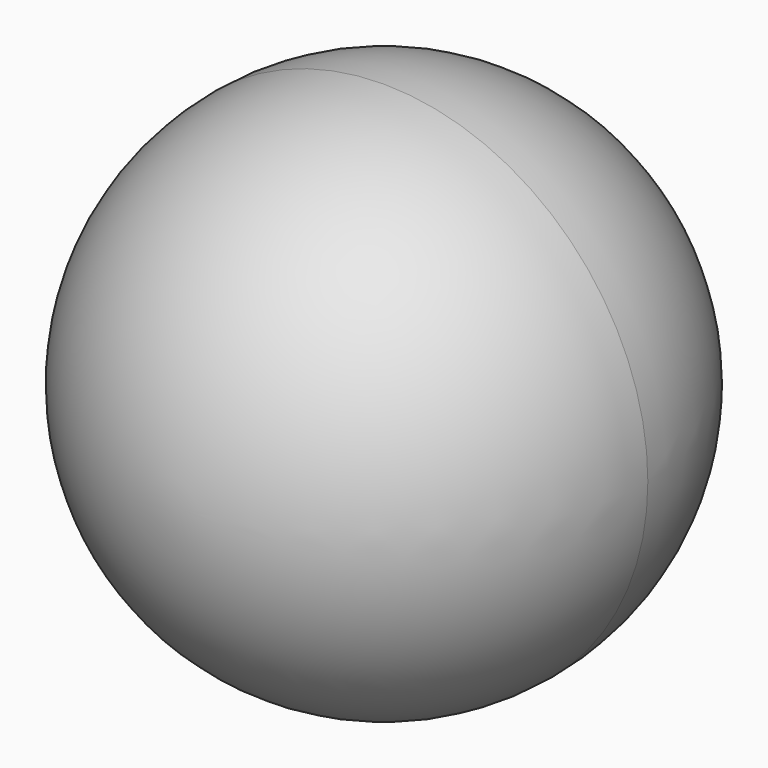
from build123d import *


with BuildPart() as f1:
    # F0 (on Top) → F1 (revolve)
    with BuildSketch(Plane.XY):
        with BuildLine():
            ThreePointArc((0, -10), (7.0710678119, -7.0710678119), (10, 0))
            ThreePointArc((10, 0), (7.0710678119, 7.0710678119), (0, 10))
            Line((0, 10), (0, 0))
            Line((0, 0), (0, -10))
        make_face()
    revolve(axis=Axis((0, 0, 0), (0, -1, 0)))


solid = f1.part
